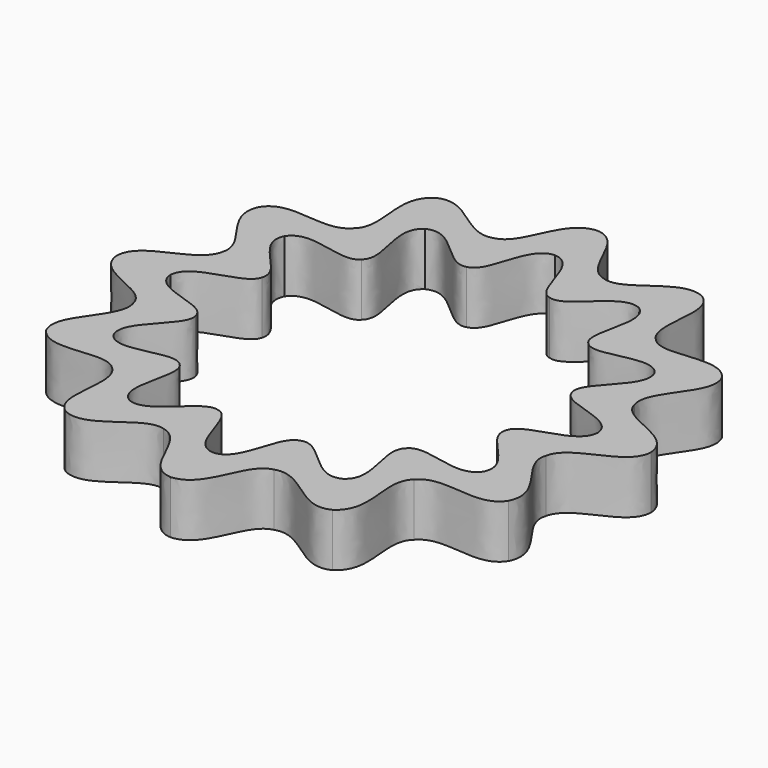
from build123d import *

# Parameters (mm, degrees)
F1_DEPTH        = 2
F1_COPIES_COUNT = 12


# Not quite as in the source:
# - a pattern or mirror of a feature is missing from the dataset's text; its kind, count and spacing are read off the source's solid


with BuildPart() as f1:
    # F0 (on Top) → F1 (new body)
    with BuildSketch(Plane.XY):
        with BuildLine():
            Line((0, 10.05), (0, 8.05))
            add(Edge.make_bspline(
                [(0, 8.05), (0.9998087881, 7.9876706484), (0.8462557502, 5.9905217807), (1.5658552229, 5.843851249)],
                knots=[0, 0, 0, 0, 2.7053640957, 2.7053640957, 2.7053640957, 2.7053640957], degree=3))
            Line((1.5658552229, 5.843851249), (2.0834933131, 7.7757029016))
            add(Edge.make_bspline(
                [(0, 10.05), (1.1240223655, 9.9869451647), (1.0816536627, 7.9769997715), (2.0834933131, 7.7757029016)],
                knots=[0, 0, 0, 0, 3.0843754112, 3.0843754112, 3.0843754112, 3.0843754112], degree=3))
        make_face()
        with BuildLine():
            Line((2.0834933131, 7.7757029016), (1.5658552229, 5.843851249))
            add(Edge.make_bspline(
                [(1.5658552229, 5.843851249), (2.3109874874, 5.5912285621), (3.1265624647, 7.4180258259), (4.025, 6.9715045005)],
                knots=[0, 0, 0, 0, 2.7053640957, 2.7053640957, 2.7053640957, 2.7053640957], degree=3))
            Line((4.025, 6.9715045005), (5.025, 8.703555308))
            add(Edge.make_bspline(
                [(2.0834933131, 7.7757029016), (2.9883467514, 7.4747764979), (3.9275781821, 9.2507637319), (5.025, 8.703555308)],
                knots=[0, 0, 0, 0, 3.0843754112, 3.0843754112, 3.0843754112, 3.0843754112], degree=3))
        make_face()
    extrude(amount=F1_DEPTH)

    # F1_copies: F1 ×12 about axis
    f1_copies_axis = Axis((0, 0, 0), (0, 0, 1))


with BuildPart() as f1_1:
    add(f1.part)
    for i in range(1, F1_COPIES_COUNT):
        add(f1.part.rotate(f1_copies_axis, i * 360 / F1_COPIES_COUNT))


solid = f1_1.part
